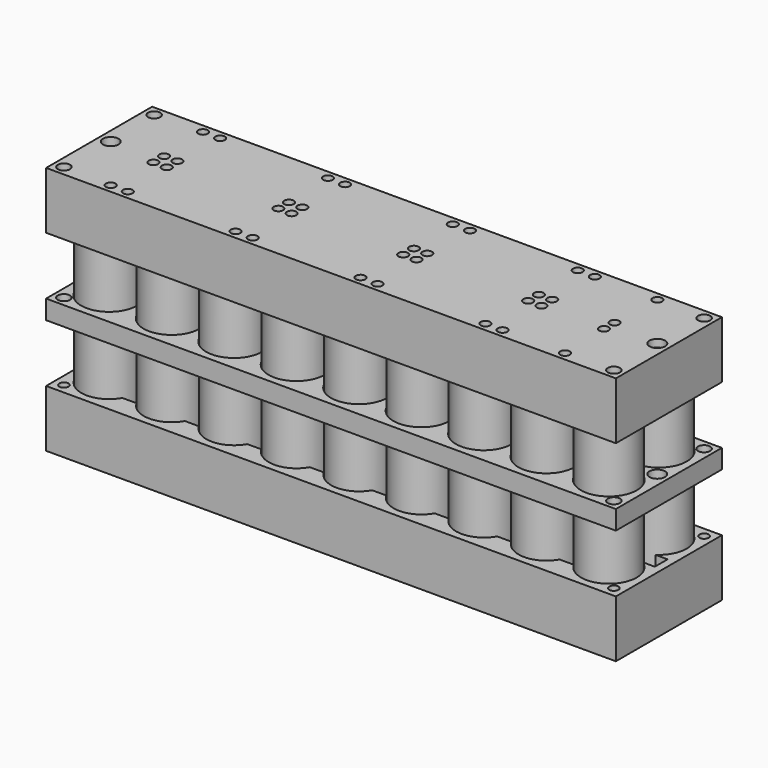
from build123d import *

# Parameters (mm, degrees)
F0_R      = 9.144
F1_DEPTH  = 65.278
F0_W      = 189.992
F0_H      = 44.196
F0_R_2    = 1.524
F0_R_3    = 6.604
F2_DEPTH  = 19.05
F0_R_4    = 2.032
F0_R_5    = 2.6035
F0_R_6    = 1.5875
F3_DEPTH  = 6.35
F4_DEPTH  = 19.05
F5_R      = 9.144
F6_DEPTH  = 10.16
F7_W      = 166.6240002223
F7_H      = 9.144
F8_DEPTH  = 16.51
F9_R      = 9.144
F10_DEPTH = 10.16
F11_W     = 167.2331261001
F11_H     = 9.144
F11_W_2   = 169.4579571486
F12_DEPTH = 16.51
F13_W     = 3.3469362922
F13_H     = 11.684
F13_W_2   = 3.3885566984
F13_H_2   = 11.8497031953
F13_W_3   = 7.5565004392
F13_H_3   = 4.9310687351
F13_W_4   = 7.5564995608
F14_DEPTH = 16.51
F15_DEPTH = 6.35
F16_W     = 18.5388238169
F16_H     = 9.144
F17_DEPTH = 16.51
F18_W     = 20.7734275609
F18_H     = 9.144
F19_DEPTH = 6.35
F20_W     = 15.8767741629
F20_H     = 11.684
F20_W_2   = 4.2492177746
F20_H_2   = 5.2381292155
F20_W_3   = 4.2999360333
F20_H_3   = 5.3398918643
F20_W_4   = 20.828
F21_DEPTH = 16.51
F22_R     = 6.604
F23_DEPTH = 2.54
F24_R     = 6.604
F25_DEPTH = 2.54
F38_R     = 9.271
F39_DEPTH = 10.16
F40_R     = 9.271
F41_DEPTH = 10.16
F42_R     = 9.271
F43_DEPTH = 10.16
F44_R     = 9.3345
F45_DEPTH = 25.4


# Not quite as in the source:
# - ends of sketch curves that miss each other by under 0.0002 mm in the source are joined


with BuildPart() as f1:
    # F0 (on Top) → F1 (new body)
    with BuildSketch(Plane.XY):
        with Locations((0, 20.828)):
            Circle(F0_R)
    extrude(amount=F1_DEPTH)

    # F16 (on face) → F17 (cut)
    with BuildSketch(Plane.XY.offset(19.05)):
        with Locations((11.1619986128, -87.3911089835)):
            Rectangle(F16_W, F16_H)
    extrude(amount=F17_DEPTH, mode=Mode.SUBTRACT)


with BuildPart() as f1b:
    # F0 (on Top) → F1, piece 2 (new body)
    with BuildSketch(Plane.XY):
        with Locations((20.828, 20.828)):
            Circle(F0_R)
    extrude(amount=F1_DEPTH)


with BuildPart() as f1c:
    # F0 (on Top) → F1, piece 3 (new body)
    with BuildSketch(Plane.XY):
        with Locations((41.656, 20.828)):
            Circle(F0_R)
    extrude(amount=F1_DEPTH)


with BuildPart() as f1d:
    # F0 (on Top) → F1, piece 4 (new body)
    with BuildSketch(Plane.XY):
        with Locations((62.484, 20.828)):
            Circle(F0_R)
    extrude(amount=F1_DEPTH)


with BuildPart() as f1e:
    # F0 (on Top) → F1, piece 5 (new body)
    with BuildSketch(Plane.XY):
        with Locations((83.312, 20.828)):
            Circle(F0_R)
    extrude(amount=F1_DEPTH)


with BuildPart() as f1f:
    # F0 (on Top) → F1, piece 6 (new body)
    with BuildSketch(Plane.XY):
        with Locations((104.14, 20.828)):
            Circle(F0_R)
    extrude(amount=F1_DEPTH)


with BuildPart() as f1g:
    # F0 (on Top) → F1, piece 7 (new body)
    with BuildSketch(Plane.XY):
        with Locations((124.968, 20.828)):
            Circle(F0_R)
    extrude(amount=F1_DEPTH)


with BuildPart() as f1h:
    # F0 (on Top) → F1, piece 8 (new body)
    with BuildSketch(Plane.XY):
        with Locations((145.796, 20.828)):
            Circle(F0_R)
    extrude(amount=F1_DEPTH)


with BuildPart() as f1i:
    # F0 (on Top) → F1, piece 9 (new body)
    with BuildSketch(Plane.XY):
        with Locations((166.624, 20.828)):
            Circle(F0_R)
    extrude(amount=F1_DEPTH)


with BuildPart() as f1j:
    # F0 (on Top) → F1, piece 10 (new body)
    with BuildSketch(Plane.XY):
        with Locations((166.624, 0)):
            Circle(F0_R)
    extrude(amount=F1_DEPTH)


with BuildPart() as f1k:
    # F0 (on Top) → F1, piece 11 (new body)
    with BuildSketch(Plane.XY):
        with Locations((145.796, 0)):
            Circle(F0_R)
    extrude(amount=F1_DEPTH)


with BuildPart() as f1l:
    # F0 (on Top) → F1, piece 12 (new body)
    with BuildSketch(Plane.XY):
        with Locations((124.968, 0)):
            Circle(F0_R)
    extrude(amount=F1_DEPTH)


with BuildPart() as f1m:
    # F0 (on Top) → F1, piece 13 (new body)
    with BuildSketch(Plane.XY):
        with Locations((104.14, 0)):
            Circle(F0_R)
    extrude(amount=F1_DEPTH)


with BuildPart() as f1n:
    # F0 (on Top) → F1, piece 14 (new body)
    with BuildSketch(Plane.XY):
        with Locations((83.312, 0)):
            Circle(F0_R)
    extrude(amount=F1_DEPTH)


with BuildPart() as f1o:
    # F0 (on Top) → F1, piece 15 (new body)
    with BuildSketch(Plane.XY):
        with Locations((62.484, 0)):
            Circle(F0_R)
    extrude(amount=F1_DEPTH)


with BuildPart() as f1p:
    # F0 (on Top) → F1, piece 16 (new body)
    with BuildSketch(Plane.XY):
        with Locations((41.656, 0)):
            Circle(F0_R)
    extrude(amount=F1_DEPTH)


with BuildPart() as f1q:
    # F0 (on Top) → F1, piece 17 (new body)
    with BuildSketch(Plane.XY):
        with Locations((20.828, 0)):
            Circle(F0_R)
    extrude(amount=F1_DEPTH)


with BuildPart() as f1r:
    # F0 (on Top) → F1, piece 18 (new body)
    with BuildSketch(Plane.XY):
        Circle(F0_R)
    extrude(amount=F1_DEPTH)


with BuildPart() as f2:
    # F0 (on Top) → F2 (new body)
    with BuildSketch(Plane.XY):
        with Locations((83.3120002223, -76.9771089835)):
            Rectangle(F0_W, F0_H)
        with Locations((-8.3819995608, -95.7731089835)):
            Circle(F0_R_2, mode=Mode.SUBTRACT)
        with Locations((2.223e-07, -87.3911089835)):
            Circle(F0_R_3, mode=Mode.SUBTRACT)
        with Locations((2.223e-07, -66.5631089835)):
            Circle(F0_R_3, mode=Mode.SUBTRACT)
        with Locations((20.8280002223, -87.3911089835)):
            Circle(F0_R_3, mode=Mode.SUBTRACT)
        with Locations((20.8280002223, -66.5631089835)):
            Circle(F0_R_3, mode=Mode.SUBTRACT)
        with Locations((-8.3819995608, -58.1811089835)):
            Circle(F0_R_2, mode=Mode.SUBTRACT)
        with Locations((41.6560002223, -87.3911089835)):
            Circle(F0_R_3, mode=Mode.SUBTRACT)
        with Locations((41.6560002223, -66.5631089835)):
            Circle(F0_R_3, mode=Mode.SUBTRACT)
        with Locations((62.4840002223, -87.3911089835)):
            Circle(F0_R_3, mode=Mode.SUBTRACT)
        with Locations((83.3120002223, -87.3911089835)):
            Circle(F0_R_3, mode=Mode.SUBTRACT)
        with Locations((62.4840002223, -66.5631089835)):
            Circle(F0_R_3, mode=Mode.SUBTRACT)
        with Locations((83.3120002223, -66.5631089835)):
            Circle(F0_R_3, mode=Mode.SUBTRACT)
        with Locations((104.1400002223, -87.3911089835)):
            Circle(F0_R_3, mode=Mode.SUBTRACT)
        with Locations((104.1400002223, -66.5631089835)):
            Circle(F0_R_3, mode=Mode.SUBTRACT)
        with Locations((124.9680002223, -87.3911089835)):
            Circle(F0_R_3, mode=Mode.SUBTRACT)
        with Locations((124.9680002223, -66.5631089835)):
            Circle(F0_R_3, mode=Mode.SUBTRACT)
        with Locations((145.7960002223, -87.3911089835)):
            Circle(F0_R_3, mode=Mode.SUBTRACT)
        with Locations((145.7960002223, -66.5631089835)):
            Circle(F0_R_3, mode=Mode.SUBTRACT)
        with Locations((175.0060004392, -95.7731089835)):
            Circle(F0_R_2, mode=Mode.SUBTRACT)
        with Locations((166.6240002223, -87.3911089835)):
            Circle(F0_R_3, mode=Mode.SUBTRACT)
        with Locations((166.6240002223, -66.5631089835)):
            Circle(F0_R_3, mode=Mode.SUBTRACT)
        with Locations((175.0060004392, -58.1811089835)):
            Circle(F0_R_2, mode=Mode.SUBTRACT)
    extrude(amount=F2_DEPTH)

    # F5 (on face) → F6 (cut)
    with BuildSketch(Plane.XY.offset(19.05)):
        with Locations((2.223e-07, -66.5631089835)):
            Circle(F5_R)
        with Locations((20.8280002223, -66.5631089835)):
            Circle(F5_R)
        with Locations((41.6560002223, -66.5631089835)):
            Circle(F5_R)
        with Locations((62.4840002223, -66.5631089835)):
            Circle(F5_R)
        with Locations((83.3120002223, -66.5631089835)):
            Circle(F5_R)
        with Locations((104.1400002223, -66.5631089835)):
            Circle(F5_R)
        with Locations((124.9680002223, -66.5631089835)):
            Circle(F5_R)
        with Locations((145.7960002223, -66.5631089835)):
            Circle(F5_R)
        with Locations((166.6240002223, -66.5631089835)):
            Circle(F5_R)
        with Locations((2.223e-07, -87.3911089835)):
            Circle(F5_R)
        with Locations((20.8280002223, -87.3911089835)):
            Circle(F5_R)
        with Locations((41.6560002223, -87.3911089835)):
            Circle(F5_R)
        with Locations((62.4840002223, -87.3911089835)):
            Circle(F5_R)
        with Locations((83.3120002223, -87.3911089835)):
            Circle(F5_R)
        with Locations((104.1400002223, -87.3911089835)):
            Circle(F5_R)
        with Locations((124.9680002223, -87.3911089835)):
            Circle(F5_R)
        with Locations((145.7960002223, -87.3911089835)):
            Circle(F5_R)
        with Locations((166.6240002223, -87.3911089835)):
            Circle(F5_R)
    extrude(amount=-F6_DEPTH, mode=Mode.SUBTRACT)

    # F7 (on face) → F8 (cut)
    with BuildSketch(Plane.XY.offset(19.05)):
        with Locations((83.3120001111, -66.5631089835)):
            Rectangle(F7_W, F7_H)
        with BuildLine():
            Line((0, -91.9631089835), (0, -82.8191089835))
            Line((0, -82.8191089835), (7.9594284191, -82.8191089835))
            ThreePointArc((7.9594284191, -82.8191089835), (-9.1790895387, -87.3911089835), (7.9594284191, -91.9631089835))
            Line((7.9594284191, -91.9631089835), (0, -91.9631089835))
        make_face()
        with BuildLine():
            Line((7.9594284191, -82.8191089835), (0, -82.8191089835))
            Line((0, -82.8191089835), (0, -91.9631089835))
            Line((0, -91.9631089835), (7.9594284191, -91.9631089835))
            ThreePointArc((7.9594284191, -91.9631089835), (8.8689342904, -89.7570526244), (9.1790895387, -87.3911089835))
            ThreePointArc((9.1790895387, -87.3911089835), (8.8689342904, -85.0251653427), (7.9594284191, -82.8191089835))
        make_face()
        with BuildLine():
            Line((166.6240002223, -82.8191089835), (7.9594284191, -82.8191089835))
            ThreePointArc((7.9594284191, -82.8191089835), (8.8689342904, -85.0251653427), (9.1790895387, -87.3911089835))
            ThreePointArc((9.1790895387, -87.3911089835), (8.8689342904, -89.7570526244), (7.9594284191, -91.9631089835))
            Line((7.9594284191, -91.9631089835), (166.6240002223, -91.9631089835))
            Line((166.6240002223, -91.9631089835), (166.6240002223, -82.8191089835))
        make_face()
    extrude(amount=-F8_DEPTH, mode=Mode.SUBTRACT)

    # F15 (add): a face of the model
    f15_faces = [f2.faces().sort_by_distance(p)[0] for p in [
        (12.0109831147, -83.1312247457, 2.54),
    ]]
    extrude(f15_faces, amount=F15_DEPTH)

    # F18 (on face) → F19 (cut)
    with BuildSketch(Plane.XY.offset(8.89)):
        with Locations((10.3867137805, -87.3911089835)):
            Rectangle(F18_W, F18_H)
    extrude(amount=-F19_DEPTH, mode=Mode.SUBTRACT)

    # F20 (on face) → F21 (cut)
    with BuildSketch(Plane.XY.offset(19.05)):
        Polygon((4.9512260593, -71.1351089835), (-4.929871764, -71.1351089835), (-4.929871764, -74.2643490264), (-4.929871764, -79.5024782419), (-4.929871764, -82.8191089835), (4.9512260593, -82.8191089835), align=None)
        with Locations((12.8896131408, -76.9771089835)):
            Rectangle(F20_W, F20_H)
        with Locations((-7.0544806514, -76.8834136342)):
            Rectangle(F20_W_2, F20_H_2)
        Polygon((171.468064189, -71.1351089835), (161.9206368923, -71.1351089835), (161.9206368923, -76.9771089835), (161.9206368923, -82.8191089835), (171.468064189, -82.8191089835), (171.468064189, -79.6585008502), (171.468064189, -74.3186089859), align=None)
        Polygon((161.9206368923, -76.9771089835), (161.9206368923, -71.1351089835), (161.9206368923, -67.7171051502), (156.2100002223, -67.7171051502), (156.2100002223, -76.9771089835), align=None)
        Polygon((161.9206368923, -82.8191089835), (161.9206368923, -76.9771089835), (156.2100002223, -76.9771089835), (156.2100002223, -87.5689461827), (161.9206368923, -87.5689461827), align=None)
        with Locations((173.6180322056, -76.988554918)):
            Rectangle(F20_W_3, F20_H_3)
        with Locations((135.3820002223, -76.9771089835)):
            Rectangle(F20_W_4, F20_H)
        with Locations((93.7260002223, -76.9771089835)):
            Rectangle(F20_W_4, F20_H)
        with Locations((52.0700002223, -76.9771089835)):
            Rectangle(F20_W_4, F20_H)
    extrude(amount=-F21_DEPTH, mode=Mode.SUBTRACT)

    # F24 (on face) → F25 (join)
    with BuildSketch(Plane(origin=(0, 0, 0), x_dir=(1, 0, 0), z_dir=(0, 0, -1))):
        with Locations((2.223e-07, 87.3911089835)):
            Circle(F24_R)
        with Locations((2.223e-07, 66.5631089835)):
            Circle(F24_R)
        with Locations((20.8280002223, 87.3911089835)):
            Circle(F24_R)
        with Locations((20.8280002223, 66.5631089835)):
            Circle(F24_R)
        with Locations((41.6560002223, 87.3911089835)):
            Circle(F24_R)
        with Locations((41.6560002223, 66.5631089835)):
            Circle(F24_R)
        with Locations((62.4840002223, 87.3911089835)):
            Circle(F24_R)
        with Locations((62.4840002223, 66.5631089835)):
            Circle(F24_R)
        with Locations((83.3120002223, 87.3911089835)):
            Circle(F24_R)
        with Locations((83.3120002223, 66.5631089835)):
            Circle(F24_R)
        with Locations((104.1400002223, 87.3911089835)):
            Circle(F24_R)
        with Locations((104.1400002223, 66.5631089835)):
            Circle(F24_R)
        with Locations((124.9680002223, 87.3911089835)):
            Circle(F24_R)
        with Locations((124.9680002223, 66.5631089835)):
            Circle(F24_R)
        with Locations((145.7960002223, 87.3911089835)):
            Circle(F24_R)
        with Locations((145.7960002223, 66.5631089835)):
            Circle(F24_R)
        with Locations((166.6240002223, 87.3911089835)):
            Circle(F24_R)
        with Locations((166.6240002223, 66.5631089835)):
            Circle(F24_R)
    extrude(amount=-F25_DEPTH)


with BuildPart() as f3:
    # F0 (on Top) → F3 (new body)
    with BuildSketch(Plane.XY):
        with Locations((83.3120002223, -138.0982894201)):
            Rectangle(F0_W, F0_H)
        with Locations((-8.3819995608, -156.8942894201)):
            Circle(F0_R_4, mode=Mode.SUBTRACT)
        with Locations((2.223e-07, -148.5122894201)):
            Circle(F0_R, mode=Mode.SUBTRACT)
        with Locations((-7.8104997777, -138.0982894201)):
            Circle(F0_R_5, mode=Mode.SUBTRACT)
        with Locations((8.1915004392, -140.3207894201)):
            Circle(F0_R_6, mode=Mode.SUBTRACT)
        with Locations((8.1915004392, -135.8757894201)):
            Circle(F0_R_6, mode=Mode.SUBTRACT)
        with Locations((20.8280002223, -148.5122894201)):
            Circle(F0_R, mode=Mode.SUBTRACT)
        with Locations((12.6365004392, -140.3207894201)):
            Circle(F0_R_6, mode=Mode.SUBTRACT)
        with Locations((12.6365004392, -135.8757894201)):
            Circle(F0_R_6, mode=Mode.SUBTRACT)
        with Locations((2.223e-07, -127.6842894201)):
            Circle(F0_R, mode=Mode.SUBTRACT)
        with Locations((-8.3819995608, -119.3022894201)):
            Circle(F0_R_4, mode=Mode.SUBTRACT)
        with Locations((20.8280002223, -127.6842894201)):
            Circle(F0_R, mode=Mode.SUBTRACT)
        with Locations((41.6560002223, -148.5122894201)):
            Circle(F0_R, mode=Mode.SUBTRACT)
        with Locations((49.8475004392, -140.3207894201)):
            Circle(F0_R_6, mode=Mode.SUBTRACT)
        with Locations((54.2925004392, -140.3207894201)):
            Circle(F0_R_6, mode=Mode.SUBTRACT)
        with Locations((49.8475004392, -135.8757894201)):
            Circle(F0_R_6, mode=Mode.SUBTRACT)
        with Locations((54.2925004392, -135.8757894201)):
            Circle(F0_R_6, mode=Mode.SUBTRACT)
        with Locations((62.4840002223, -148.5122894201)):
            Circle(F0_R, mode=Mode.SUBTRACT)
        with Locations((83.3120002223, -148.5122894201)):
            Circle(F0_R, mode=Mode.SUBTRACT)
        with Locations((41.6560002223, -127.6842894201)):
            Circle(F0_R, mode=Mode.SUBTRACT)
        with Locations((62.4840002223, -127.6842894201)):
            Circle(F0_R, mode=Mode.SUBTRACT)
        with Locations((83.3120002223, -127.6842894201)):
            Circle(F0_R, mode=Mode.SUBTRACT)
        with Locations((104.1400002223, -148.5122894201)):
            Circle(F0_R, mode=Mode.SUBTRACT)
        with Locations((91.5035004392, -140.3207894201)):
            Circle(F0_R_6, mode=Mode.SUBTRACT)
        with Locations((91.5035004392, -135.8757894201)):
            Circle(F0_R_6, mode=Mode.SUBTRACT)
        with Locations((95.9485004392, -140.3207894201)):
            Circle(F0_R_6, mode=Mode.SUBTRACT)
        with Locations((95.9485004392, -135.8757894201)):
            Circle(F0_R_6, mode=Mode.SUBTRACT)
        with Locations((124.9680002223, -148.5122894201)):
            Circle(F0_R, mode=Mode.SUBTRACT)
        with Locations((104.1400002223, -127.6842894201)):
            Circle(F0_R, mode=Mode.SUBTRACT)
        with Locations((124.9680002223, -127.6842894201)):
            Circle(F0_R, mode=Mode.SUBTRACT)
        with Locations((145.7960002223, -148.5122894201)):
            Circle(F0_R, mode=Mode.SUBTRACT)
        with Locations((133.1595004392, -140.3207894201)):
            Circle(F0_R_6, mode=Mode.SUBTRACT)
        with Locations((137.6045004392, -140.3207894201)):
            Circle(F0_R_6, mode=Mode.SUBTRACT)
        with Locations((133.1595004392, -135.8757894201)):
            Circle(F0_R_6, mode=Mode.SUBTRACT)
        with Locations((137.6045004392, -135.8757894201)):
            Circle(F0_R_6, mode=Mode.SUBTRACT)
        with Locations((175.0060004392, -156.8942894201)):
            Circle(F0_R_4, mode=Mode.SUBTRACT)
        with Locations((166.6240002223, -148.5122894201)):
            Circle(F0_R, mode=Mode.SUBTRACT)
        with Locations((158.4325004392, -140.3207894201)):
            Circle(F0_R_6, mode=Mode.SUBTRACT)
        with Locations((158.4325004392, -135.8757894201)):
            Circle(F0_R_6, mode=Mode.SUBTRACT)
        with Locations((174.4345002223, -138.0982894201)):
            Circle(F0_R_5, mode=Mode.SUBTRACT)
        with Locations((145.7960002223, -127.6842894201)):
            Circle(F0_R, mode=Mode.SUBTRACT)
        with Locations((166.6240002223, -127.6842894201)):
            Circle(F0_R, mode=Mode.SUBTRACT)
        with Locations((175.0060004392, -119.3022894201)):
            Circle(F0_R_4, mode=Mode.SUBTRACT)
    extrude(amount=F3_DEPTH)


with BuildPart() as f4:
    # F0 (on Top) → F4 (new body)
    with BuildSketch(Plane.XY):
        with Locations((83.3120004392, -204.8083442945)):
            Rectangle(F0_W, F0_H)
        with Locations((-8.3819995608, -223.6043442945)):
            Circle(F0_R_4, mode=Mode.SUBTRACT)
        with Locations((4.392e-07, -215.2223442945)):
            Circle(F0_R_3, mode=Mode.SUBTRACT)
        with Locations((7.5565004392, -224.0488442945)):
            Circle(F0_R_6, mode=Mode.SUBTRACT)
        with Locations((-7.8104995608, -204.8083442945)):
            Circle(F0_R_5, mode=Mode.SUBTRACT)
        with Locations((8.1915004392, -207.0308442945)):
            Circle(F0_R_6, mode=Mode.SUBTRACT)
        with Locations((8.1915004392, -202.5858442945)):
            Circle(F0_R_6, mode=Mode.SUBTRACT)
        with Locations((13.2715004392, -224.0488442945)):
            Circle(F0_R_6, mode=Mode.SUBTRACT)
        with Locations((20.8280004392, -215.2223442945)):
            Circle(F0_R_3, mode=Mode.SUBTRACT)
        with Locations((12.6365004392, -207.0308442945)):
            Circle(F0_R_6, mode=Mode.SUBTRACT)
        with Locations((12.6365004392, -202.5858442945)):
            Circle(F0_R_6, mode=Mode.SUBTRACT)
        with Locations((4.392e-07, -194.3943442945)):
            Circle(F0_R_3, mode=Mode.SUBTRACT)
        with Locations((-8.3819995608, -186.0123442945)):
            Circle(F0_R_4, mode=Mode.SUBTRACT)
        with Locations((7.5565004392, -185.5678442945)):
            Circle(F0_R_6, mode=Mode.SUBTRACT)
        with Locations((20.8280004392, -194.3943442945)):
            Circle(F0_R_3, mode=Mode.SUBTRACT)
        with Locations((13.2715004392, -185.5678442945)):
            Circle(F0_R_6, mode=Mode.SUBTRACT)
        with Locations((41.6560004392, -215.2223442945)):
            Circle(F0_R_3, mode=Mode.SUBTRACT)
        with Locations((49.2125004392, -224.0488442945)):
            Circle(F0_R_6, mode=Mode.SUBTRACT)
        with Locations((54.9275004392, -224.0488442945)):
            Circle(F0_R_6, mode=Mode.SUBTRACT)
        with Locations((49.8475004392, -207.0308442945)):
            Circle(F0_R_6, mode=Mode.SUBTRACT)
        with Locations((54.2925004392, -207.0308442945)):
            Circle(F0_R_6, mode=Mode.SUBTRACT)
        with Locations((49.8475004392, -202.5858442945)):
            Circle(F0_R_6, mode=Mode.SUBTRACT)
        with Locations((54.2925004392, -202.5858442945)):
            Circle(F0_R_6, mode=Mode.SUBTRACT)
        with Locations((62.4840004392, -215.2223442945)):
            Circle(F0_R_3, mode=Mode.SUBTRACT)
        with Locations((41.6560004392, -194.3943442945)):
            Circle(F0_R_3, mode=Mode.SUBTRACT)
        with Locations((49.2125004392, -185.5678442945)):
            Circle(F0_R_6, mode=Mode.SUBTRACT)
        with Locations((54.9275004392, -185.5678442945)):
            Circle(F0_R_6, mode=Mode.SUBTRACT)
        with Locations((62.4840004392, -194.3943442945)):
            Circle(F0_R_3, mode=Mode.SUBTRACT)
        with Locations((90.8685004392, -224.0488442945)):
            Circle(F0_R_6, mode=Mode.SUBTRACT)
        with Locations((83.3120004392, -215.2223442945)):
            Circle(F0_R_3, mode=Mode.SUBTRACT)
        with Locations((96.5835004392, -224.0488442945)):
            Circle(F0_R_6, mode=Mode.SUBTRACT)
        with Locations((104.1400004392, -215.2223442945)):
            Circle(F0_R_3, mode=Mode.SUBTRACT)
        with Locations((91.5035004392, -207.0308442945)):
            Circle(F0_R_6, mode=Mode.SUBTRACT)
        with Locations((91.5035004392, -202.5858442945)):
            Circle(F0_R_6, mode=Mode.SUBTRACT)
        with Locations((95.9485004392, -207.0308442945)):
            Circle(F0_R_6, mode=Mode.SUBTRACT)
        with Locations((95.9485004392, -202.5858442945)):
            Circle(F0_R_6, mode=Mode.SUBTRACT)
        with Locations((124.9680004392, -215.2223442945)):
            Circle(F0_R_3, mode=Mode.SUBTRACT)
        with Locations((83.3120004392, -194.3943442945)):
            Circle(F0_R_3, mode=Mode.SUBTRACT)
        with Locations((90.8685004392, -185.5678442945)):
            Circle(F0_R_6, mode=Mode.SUBTRACT)
        with Locations((104.1400004392, -194.3943442945)):
            Circle(F0_R_3, mode=Mode.SUBTRACT)
        with Locations((96.5835004392, -185.5678442945)):
            Circle(F0_R_6, mode=Mode.SUBTRACT)
        with Locations((124.9680004392, -194.3943442945)):
            Circle(F0_R_3, mode=Mode.SUBTRACT)
        with Locations((132.5245004392, -224.0488442945)):
            Circle(F0_R_6, mode=Mode.SUBTRACT)
        with Locations((138.2395004392, -224.0488442945)):
            Circle(F0_R_6, mode=Mode.SUBTRACT)
        with Locations((145.7960004392, -215.2223442945)):
            Circle(F0_R_3, mode=Mode.SUBTRACT)
        with Locations((133.1595004392, -207.0308442945)):
            Circle(F0_R_6, mode=Mode.SUBTRACT)
        with Locations((137.6045004392, -207.0308442945)):
            Circle(F0_R_6, mode=Mode.SUBTRACT)
        with Locations((133.1595004392, -202.5858442945)):
            Circle(F0_R_6, mode=Mode.SUBTRACT)
        with Locations((137.6045004392, -202.5858442945)):
            Circle(F0_R_6, mode=Mode.SUBTRACT)
        with Locations((159.0675004392, -224.0488442945)):
            Circle(F0_R_6, mode=Mode.SUBTRACT)
        with Locations((175.0060004392, -223.6043442945)):
            Circle(F0_R_4, mode=Mode.SUBTRACT)
        with Locations((166.6240004392, -215.2223442945)):
            Circle(F0_R_3, mode=Mode.SUBTRACT)
        with Locations((158.4325004392, -207.0308442945)):
            Circle(F0_R_6, mode=Mode.SUBTRACT)
        with Locations((158.4325004392, -202.5858442945)):
            Circle(F0_R_6, mode=Mode.SUBTRACT)
        with Locations((174.4345004392, -204.8083442945)):
            Circle(F0_R_5, mode=Mode.SUBTRACT)
        with Locations((132.5245004392, -185.5678442945)):
            Circle(F0_R_6, mode=Mode.SUBTRACT)
        with Locations((138.2395004392, -185.5678442945)):
            Circle(F0_R_6, mode=Mode.SUBTRACT)
        with Locations((145.7960004392, -194.3943442945)):
            Circle(F0_R_3, mode=Mode.SUBTRACT)
        with Locations((159.0675004392, -185.5678442945)):
            Circle(F0_R_6, mode=Mode.SUBTRACT)
        with Locations((166.6240004392, -194.3943442945)):
            Circle(F0_R_3, mode=Mode.SUBTRACT)
        with Locations((175.0060004392, -186.0123442945)):
            Circle(F0_R_4, mode=Mode.SUBTRACT)
    extrude(amount=F4_DEPTH)

    # F9 (on face) → F10 (cut)
    with BuildSketch(Plane(origin=(0, 0, 0), x_dir=(1, 0, 0), z_dir=(0, 0, -1))):
        with Locations((4.392e-07, 215.2223442945)):
            Circle(F9_R)
        with Locations((20.8280004392, 215.2223442945)):
            Circle(F9_R)
        with Locations((41.6560004392, 215.2223442945)):
            Circle(F9_R)
        with Locations((62.4840004392, 215.2223442945)):
            Circle(F9_R)
        with Locations((83.3120004392, 215.2223442945)):
            Circle(F9_R)
        with Locations((104.1400004392, 215.2223442945)):
            Circle(F9_R)
        with Locations((124.9680004392, 215.2223442945)):
            Circle(F9_R)
        with Locations((145.7960004392, 215.2223442945)):
            Circle(F9_R)
        with Locations((166.6240004392, 215.2223442945)):
            Circle(F9_R)
        with Locations((4.392e-07, 194.3943442945)):
            Circle(F9_R)
        with Locations((20.8280004392, 194.3943442945)):
            Circle(F9_R)
        with Locations((41.6560004392, 194.3943442945)):
            Circle(F9_R)
        with Locations((62.4840004392, 194.3943442945)):
            Circle(F9_R)
        with Locations((83.3120004392, 194.3943442945)):
            Circle(F9_R)
        with Locations((104.1400004392, 194.3943442945)):
            Circle(F9_R)
        with Locations((124.9680004392, 194.3943442945)):
            Circle(F9_R)
        with Locations((145.7960004392, 194.3943442945)):
            Circle(F9_R)
        with Locations((166.6240004392, 194.3943442945)):
            Circle(F9_R)
    extrude(amount=-F10_DEPTH, mode=Mode.SUBTRACT)

    # F11 (on face) → F12 (cut)
    with BuildSketch(Plane(origin=(0, 0, 0), x_dir=(1, 0, 0), z_dir=(0, 0, -1))):
        with Locations((83.61656305, 215.2223442945)):
            Rectangle(F11_W, F11_H)
        with Locations((84.7289785743, 194.3943442945)):
            Rectangle(F11_W_2, F11_H)
    extrude(amount=-F12_DEPTH, mode=Mode.SUBTRACT)

    # F13 (on face) → F14 (cut)
    with BuildSketch(Plane(origin=(0, 0, 0), x_dir=(1, 0, 0), z_dir=(0, 0, -1))):
        Polygon((171.1960004392, 214.9480893754), (162.0520004392, 214.9480893754), (162.0520004392, 194.13798903), (171.1960004392, 194.13798903), (171.1960004392, 198.9663442945), (171.1960004392, 210.6503442945), align=None)
        with Locations((172.8694685853, 204.8083442945)):
            Rectangle(F13_W, F13_H)
        Polygon((4.5720004392, 215.7430916327), (-4.5719995608, 215.7430916327), (-4.5719995608, 210.743188858), (-4.5719995608, 198.8934856627), (-4.5719995608, 194.13798903), (4.5720004392, 194.13798903), align=None)
        with Locations((-6.26627791, 204.8183372604)):
            Rectangle(F13_W_2, F13_H_2)
        with Locations((3.7782502196, 221.583309927)):
            Rectangle(F13_W_3, F13_H_3)
        with Locations((3.7782502196, 188.0333786621)):
            Rectangle(F13_W_3, F13_H_3)
        with Locations((17.0497506588, 221.583309927)):
            Rectangle(F13_W_3, F13_H_3)
        with Locations((17.0497506588, 188.0333786621)):
            Rectangle(F13_W_3, F13_H_3)
        Polygon((49.2125004392, 224.0488442945), (41.656, 224.0488442945), (41.6560008785, 219.1177755594), (49.2125004392, 219.1177755594), align=None)
        with Locations((45.4342506588, 188.0333786621)):
            Rectangle(F13_W_4, F13_H_3)
        with Locations((58.7057506588, 221.583309927)):
            Rectangle(F13_W_3, F13_H_3)
        with Locations((58.7057506588, 188.0333786621)):
            Rectangle(F13_W_3, F13_H_3)
        Polygon((90.8685004392, 224.0488442945), (83.312, 224.0488442945), (83.3120008785, 219.1177755594), (90.8685004392, 219.1177755594), align=None)
        with Locations((79.5337506588, 188.0333786621)):
            Rectangle(F13_W_3, F13_H_3)
        Polygon((90.8685004392, 190.4989130297), (83.312, 190.4989130297), (83.3120008785, 185.5678442945), (90.8685004392, 185.5678442945), align=None)
        with Locations((100.3617506588, 221.583309927)):
            Rectangle(F13_W_3, F13_H_3)
        with Locations((100.3617506588, 188.0333786621)):
            Rectangle(F13_W_3, F13_H_3)
        Polygon((132.5245004392, 224.0488442945), (124.968, 224.0488442945), (124.9680008785, 219.1177755594), (132.5245004392, 219.1177755594), align=None)
        with Locations((128.7462506588, 188.0333786621)):
            Rectangle(F13_W_4, F13_H_3)
        with Locations((142.0177506588, 221.583309927)):
            Rectangle(F13_W_3, F13_H_3)
        with Locations((142.0177506588, 188.0333786621)):
            Rectangle(F13_W_3, F13_H_3)
        with Locations((162.8457506588, 221.583309927)):
            Rectangle(F13_W_3, F13_H_3)
        with Locations((162.8457506588, 188.0333786621)):
            Rectangle(F13_W_3, F13_H_3)
    extrude(amount=-F14_DEPTH, mode=Mode.SUBTRACT)

    # F22 (on face) → F23 (join)
    with BuildSketch(Plane.XY.offset(19.05)):
        with Locations((4.392e-07, -194.3943442945)):
            Circle(F22_R)
        with Locations((4.392e-07, -215.2223442945)):
            Circle(F22_R)
        with Locations((20.8280004392, -194.3943442945)):
            Circle(F22_R)
        with Locations((20.8280004392, -215.2223442945)):
            Circle(F22_R)
        with Locations((41.6560004392, -194.3943442945)):
            Circle(F22_R)
        with Locations((41.6560004392, -215.2223442945)):
            Circle(F22_R)
        with Locations((62.4840004392, -194.3943442945)):
            Circle(F22_R)
        with Locations((62.4840004392, -215.2223442945)):
            Circle(F22_R)
        with Locations((83.3120004392, -194.3943442945)):
            Circle(F22_R)
        with Locations((83.3120004392, -215.2223442945)):
            Circle(F22_R)
        with Locations((104.1400004392, -194.3943442945)):
            Circle(F22_R)
        with Locations((104.1400004392, -215.2223442945)):
            Circle(F22_R)
        with Locations((124.9680004392, -194.3943442945)):
            Circle(F22_R)
        with Locations((124.9680004392, -215.2223442945)):
            Circle(F22_R)
        with Locations((145.7960004392, -194.3943442945)):
            Circle(F22_R)
        with Locations((145.7960004392, -215.2223442945)):
            Circle(F22_R)
        with Locations((166.6240004392, -194.3943442945)):
            Circle(F22_R)
        with Locations((166.6240004392, -215.2223442945)):
            Circle(F22_R)
    extrude(amount=-F23_DEPTH)


with BuildPart() as f4_1:
    # F26: moved
    add(f4.part.moved(Location((0, 127.8382, 44.958))))


with BuildPart() as f3_1:
    # F27: moved
    add(f3.part.moved(Location((0, 61.1124, 22.733))))


with BuildPart() as f2_1:
    # F28: moved
    add(f2.part.moved(Location((0, 0, -8.89))))


with BuildPart() as f2_2:
    # F29: moved
    add(f2_1.part.moved(Location((0, 0, 8.89))))


with BuildPart() as f3_2:
    # F29: moved
    add(f3_1.part.moved(Location((0, 0, 8.89))))


with BuildPart() as f4_2:
    # F29: moved
    add(f4_1.part.moved(Location((0, 0, 8.89))))


with BuildPart() as f2_3:
    # F30: moved
    add(f2_2.part.moved(Location((0, 87.4268, 0))))


with BuildPart() as f3_3:
    # F31: moved
    add(f3_2.part.moved(Location((0, 87.4268, 0))))


with BuildPart() as f4_3:
    # F32: moved
    add(f4_2.part.moved(Location((0, 87.4268, 0))))


with BuildPart() as f2_4:
    # F33: moved
    add(f2_3.part.moved(Location((0, 0, -2.54))))


with BuildPart() as f2_5:
    # F34: moved
    add(f2_4.part.moved(Location((0, 0, -6.35))))


with BuildPart() as f4_4:
    # F35: moved
    add(f4_3.part.moved(Location((0, 0, 1.27))))

    # F38 (on face) → F39 (cut)
    with BuildSketch(Plane(origin=(0, 0, 55.118), x_dir=(1, 0, 0), z_dir=(0, 0, -1))):
        with Locations((166.6240004392, -20.8706557055)):
            Circle(F38_R)
        with Locations((166.6240004392, -0.0426557055)):
            Circle(F38_R)
        with Locations((145.7960004392, -20.8706557055)):
            Circle(F38_R)
        with Locations((145.7960004392, -0.0426557055)):
            Circle(F38_R)
        with Locations((124.9680004392, -20.8706557055)):
            Circle(F38_R)
        with Locations((124.9680004392, -0.0426557055)):
            Circle(F38_R)
        with Locations((104.1400004392, -20.8706557055)):
            Circle(F38_R)
        with Locations((104.1400004392, -0.0426557055)):
            Circle(F38_R)
        with Locations((83.3120004392, -20.8706557055)):
            Circle(F38_R)
        with Locations((83.3120004392, -0.0426557055)):
            Circle(F38_R)
        with Locations((62.4840004392, -20.8706557055)):
            Circle(F38_R)
        with Locations((62.4840004392, -0.0426557055)):
            Circle(F38_R)
        with Locations((41.6560004392, -20.8706557055)):
            Circle(F38_R)
        with Locations((41.6560004392, -0.0426557055)):
            Circle(F38_R)
        with Locations((20.8280004392, -20.8706557055)):
            Circle(F38_R)
        with Locations((20.8280004392, -0.0426557055)):
            Circle(F38_R)
        with Locations((4.392e-07, -20.8706557055)):
            Circle(F38_R)
        with Locations((4.392e-07, -0.0426557055)):
            Circle(F38_R)
    extrude(amount=-F39_DEPTH, mode=Mode.SUBTRACT)


with BuildPart() as f2_6:
    # F35: moved
    add(f2_5.part.moved(Location((0, 0, 1.27))))


with BuildPart() as f2_7:
    # F36: moved
    add(f2_6.part.moved(Location((0, 0, -1.27))))

    # F40 (on face) → F41 (cut)
    with BuildSketch(Plane.XY.offset(10.16)):
        with Locations((166.6240002223, 0.0356910165)):
            Circle(F40_R)
        with Locations((166.6240002223, 20.8636910165)):
            Circle(F40_R)
        with Locations((145.7960002223, 0.0356910165)):
            Circle(F40_R)
        with Locations((145.7960002223, 20.8636910165)):
            Circle(F40_R)
        with Locations((124.9680002223, 0.0356910165)):
            Circle(F40_R)
        with Locations((124.9680002223, 20.8636910165)):
            Circle(F40_R)
        with Locations((104.1400002223, 0.0356910165)):
            Circle(F40_R)
        with Locations((104.1400002223, 20.8636910165)):
            Circle(F40_R)
        with Locations((83.3120002223, 0.0356910165)):
            Circle(F40_R)
        with Locations((83.3120002223, 20.8636910165)):
            Circle(F40_R)
        with Locations((62.4840002223, 0.0356910165)):
            Circle(F40_R)
        with Locations((62.4840002223, 20.8636910165)):
            Circle(F40_R)
        with Locations((41.6560002223, 0.0356910165)):
            Circle(F40_R)
        with Locations((41.6560002223, 20.8636910165)):
            Circle(F40_R)
        with Locations((20.8280002223, 0.0356910165)):
            Circle(F40_R)
        with Locations((20.8280002223, 20.8636910165)):
            Circle(F40_R)
        with Locations((2.223e-07, 0.0356910165)):
            Circle(F40_R)
        with Locations((2.223e-07, 20.8636910165)):
            Circle(F40_R)
    extrude(amount=-F41_DEPTH, mode=Mode.SUBTRACT)


with BuildPart() as f3_4:
    # F37: moved
    add(f3_3.part.moved(Location((0, 0, -2.159))))

    # F42 (on face) → F43 (cut)
    with BuildSketch(Plane.XY.offset(35.814)):
        with Locations((166.6240002223, 0.0269105799)):
            Circle(F42_R)
        with Locations((166.6240002223, 20.8549105799)):
            Circle(F42_R)
        with Locations((145.7960002223, 0.0269105799)):
            Circle(F42_R)
        with Locations((145.7960002223, 20.8549105799)):
            Circle(F42_R)
        with Locations((124.9680002223, 0.0269105799)):
            Circle(F42_R)
        with Locations((124.9680002223, 20.8549105799)):
            Circle(F42_R)
        with Locations((104.1400002223, 0.0269105799)):
            Circle(F42_R)
        with Locations((104.1400002223, 20.8549105799)):
            Circle(F42_R)
        with Locations((83.3120002223, 0.0269105799)):
            Circle(F42_R)
        with Locations((83.3120002223, 20.8549105799)):
            Circle(F42_R)
        with Locations((62.4840002223, 0.0269105799)):
            Circle(F42_R)
        with Locations((62.4840002223, 20.8549105799)):
            Circle(F42_R)
        with Locations((41.6560002223, 0.0269105799)):
            Circle(F42_R)
        with Locations((41.6560002223, 20.8549105799)):
            Circle(F42_R)
        with Locations((20.8280002223, 0.0269105799)):
            Circle(F42_R)
        with Locations((20.8280002223, 20.8549105799)):
            Circle(F42_R)
        with Locations((2.223e-07, 0.0269105799)):
            Circle(F42_R)
        with Locations((2.223e-07, 20.8549105799)):
            Circle(F42_R)
    extrude(amount=-F43_DEPTH, mode=Mode.SUBTRACT)

    # F44 (on face) → F45 (cut)
    with BuildSketch(Plane.XY.offset(35.814)):
        with Locations((2.223e-07, 20.8549105799)):
            Circle(F44_R)
        with Locations((2.223e-07, 0.0269105799)):
            Circle(F44_R)
        with Locations((20.8280002223, 20.8549105799)):
            Circle(F44_R)
        with Locations((20.8280002223, 0.0269105799)):
            Circle(F44_R)
        with Locations((41.6560002223, 20.8549105799)):
            Circle(F44_R)
        with Locations((41.6560002223, 0.0269105799)):
            Circle(F44_R)
        with Locations((62.4840002223, 20.8549105799)):
            Circle(F44_R)
        with Locations((62.4840002223, 0.0269105799)):
            Circle(F44_R)
        with Locations((83.3120002223, 20.8549105799)):
            Circle(F44_R)
        with Locations((83.3120002223, 0.0269105799)):
            Circle(F44_R)
        with Locations((104.1400002223, 20.8549105799)):
            Circle(F44_R)
        with Locations((104.1400002223, 0.0269105799)):
            Circle(F44_R)
        with Locations((124.9680002223, 20.8549105799)):
            Circle(F44_R)
        with Locations((124.9680002223, 0.0269105799)):
            Circle(F44_R)
        with Locations((145.7960002223, 20.8549105799)):
            Circle(F44_R)
        with Locations((145.7960002223, 0.0269105799)):
            Circle(F44_R)
        with Locations((166.6240002223, 20.8549105799)):
            Circle(F44_R)
        with Locations((166.6240002223, 0.0269105799)):
            Circle(F44_R)
    extrude(amount=-F45_DEPTH, mode=Mode.SUBTRACT)


solid = Compound([f1.part, f1b.part, f1c.part, f1d.part, f1e.part, f1f.part, f1g.part, f1h.part, f1i.part, f1j.part, f1k.part, f1l.part, f1m.part, f1n.part, f1o.part, f1p.part, f1q.part, f1r.part, f4_4.part, f2_7.part, f3_4.part])
